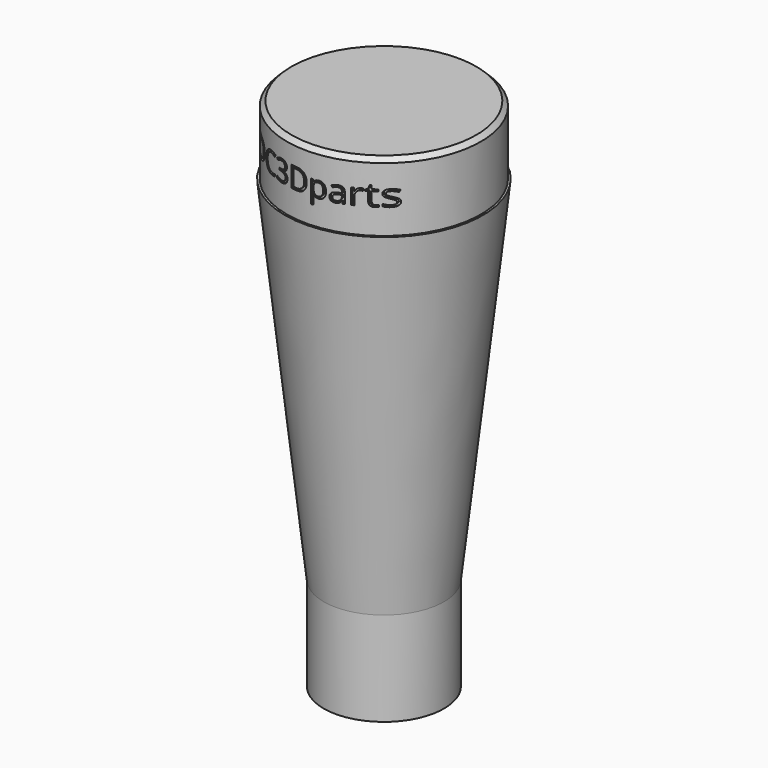
from build123d import *

# Parameters (mm, degrees)
F2_SIZE      = 1.5
F4_TEXT_SIZE = 9.7222222222
F5_DEPTH     = 40
F6_W         = 32
F6_H         = 24.557184213


# Not quite as in the source:
# - Text() gives the source's letters only with a copy of the font that has no kerning and outlines rounded to 1/6400 em; it was checked with that copy


with BuildPart() as f1:
    # F0 (on Front) → F1 (revolve)
    with BuildSketch(Plane.XZ):
        Polygon((0, 66.2666279856), (-32.55, 66.2666279856), (-32.55, 43.2666279856), (-33.25, 43.2666279856), (-20.2, -75.179155147), (-20.2, -106.7333720144), (0, -106.7333720144), align=None)
    revolve(axis=Axis((0, 0, -2.5966958965), (0, 0, -1)))

    # F2
    f2_edges = [f1.edges().sort_by_distance(p)[0] for p in [
        (32.55, 0, 66.266628),
    ]]
    chamfer(f2_edges, length=F2_SIZE)


with BuildPart() as f5:
    # F4 (on offset) → F5 (new body, through all)
    with BuildSketch(Plane.XZ.offset(40)):
        with Locations((-25.1410925611, 51.8211234414)):
            Text('DC3Dparts', F4_TEXT_SIZE, font='Open Sans', text_align=(TextAlign.LEFT, TextAlign.BOTTOM))
    extrude(amount=-F5_DEPTH)


with BuildPart() as f7:
    # F6 (on Front) → F7 (revolve)
    with BuildSketch(Plane.XZ):
        with Locations((-16, 59.0576304638)):
            Rectangle(F6_W, F6_H)
    revolve(axis=Axis((0, 0, 59.0576304638), (0, 0, 1)))


with BuildPart() as f5_1:
    add(f5.part)

    # F8: cut F7
    add(f7.part, mode=Mode.SUBTRACT)


with BuildPart() as f1_1:
    add(f1.part)

    # F9: cut F5
    add(f5_1.part, mode=Mode.SUBTRACT)


solid = f1_1.part
